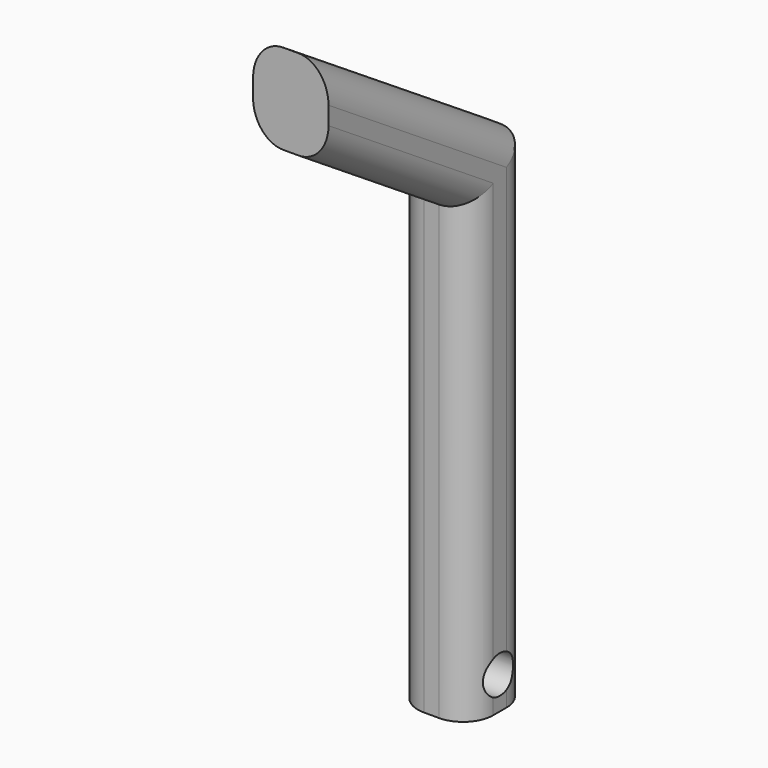
from build123d import *

# Parameters (mm, degrees)
F0_R         = 3.175
F1_DEPTH     = 12.7
F3_DEPTH     = 12.701
F4_T1_DEPTH  = 108.2499657273
F4_T3_DEPTH  = 76.2
F4_T8_DEPTH  = 101.5317029417
F4_T13_DEPTH = 101.5317029417
F4_T18_DEPTH = 60.7438000865
F4_T23_DEPTH = 60.7438000865
F4_T29_DEPTH = 101.5317029417
F4_T33_DEPTH = 60.7438000865
F4_T40_DEPTH = 101.5317029417
F4_T44_DEPTH = 60.7438000865


# Not quite as in the source:
# - a fillet or chamfer that OpenCascade refuses, or shapes differently, is made with other operations: its cross-section is extruded or revolved along the edge and cut away or added


with BuildPart() as f1:
    # F0 (on Right) → F1 (new body)
    with BuildSketch(Plane.YZ):
        Polygon((-12.9443686455, 18.7500342727), (0, 18.7500342727), (0, 101.6), (-42.5443466617, 129.3600174195), (-49.4843510166, 118.7239307541), (-12.9443686455, 94.8817372144), align=None)
        with Locations((-6.4721843228, 24.2384169251)):
            Circle(F0_R, mode=Mode.SUBTRACT)
    extrude(amount=F1_DEPTH)

    # F2 (on face) → F3 (cut, through all)
    with BuildSketch(Plane(origin=(0, 0, 0), x_dir=(0, -1, 0), z_dir=(-1, 0, 0))):
        Polygon((49.4843510166, 118.7239307541), (42.5443466617, 129.3600174195), (42.5443466617, 114.1956054441), align=None)
    extrude(amount=-F3_DEPTH, mode=Mode.SUBTRACT)

    # F4: fillet of radius 5.08 on 8 edges, made by hand

    # F4_s2 → F4_t1 (cut)
    with BuildSketch(Plane.XY.offset(6.0500342727)):
        with BuildLine():
            ThreePointArc((0, -5.08), (1.4878975516, -1.4878975516), (5.08, 0))
            Line((5.08, 0), (0, 0))
            Line((0, 0), (0, -5.08))
        make_face()
        with BuildLine():
            ThreePointArc((12.7, -5.08), (11.2121024484, -1.4878975516), (7.62, 0))
            Line((7.62, 0), (12.7, 0))
            Line((12.7, 0), (12.7, -5.08))
        make_face()
    extrude(amount=F4_T1_DEPTH, mode=Mode.SUBTRACT)

    # F4_s4 → F4_t3 (cut)
    with BuildSketch(Plane(origin=(0, -35.8612284696, 23.3993093117), x_dir=(1, 0, 0), z_dir=(0, -0.837487139, 0.5464570358))):
        with BuildLine():
            ThreePointArc((12.7, 80.0086933233), (11.2121024484, 83.6007957718), (7.62, 85.0886933233))
            Line((7.62, 85.0886933233), (12.7, 85.0886933233))
            Line((12.7, 85.0886933233), (12.7, 80.0086933233))
        make_face()
        with BuildLine():
            ThreePointArc((0, 80.0086933233), (1.4878975516, 83.6007957718), (5.08, 85.0886933233))
            Line((5.08, 85.0886933233), (0, 85.0886933233))
            Line((0, 85.0886933233), (0, 80.0086933233))
        make_face()
    extrude(amount=F4_T3_DEPTH, mode=Mode.SUBTRACT)


with BuildPart() as f4_tool6:
    # F4_s7 → F4_t8 (new body)
    with BuildSketch(Plane.XY.offset(107.5817372144)):
        with BuildLine():
            ThreePointArc((5.08, -12.9443686455), (1.4878975516, -11.456471094), (0, -7.8643686455))
            Line((0, -7.8643686455), (0, -12.9443686455))
            Line((0, -12.9443686455), (5.08, -12.9443686455))
        make_face()
    extrude(amount=-F4_T8_DEPTH)

    split(bisect_by=Plane(origin=(0, 39.5573107801, 60.624599668), x_dir=(1, 0, 0), z_dir=(0, -0.5464570358, -0.837487139)), keep=Keep.TOP)


with BuildPart() as f1_1:
    add(f1.part)

    # F4_t5: cut F4_tool6
    add(f4_tool6.part, mode=Mode.SUBTRACT)


with BuildPart() as f4_tool11:
    # F4_s12 → F4_t13 (new body)
    with BuildSketch(Plane.XY.offset(107.5817372144)):
        with BuildLine():
            ThreePointArc((7.62, -12.9443686455), (11.2121024484, -11.456471094), (12.7, -7.8643686455))
            Line((12.7, -7.8643686455), (12.7, -12.9443686455))
            Line((12.7, -12.9443686455), (7.62, -12.9443686455))
        make_face()
    extrude(amount=-F4_T13_DEPTH)

    split(bisect_by=Plane(origin=(0, 39.5573107801, 60.624599668), x_dir=(1, 0, 0), z_dir=(0, -0.5464570358, -0.837487139)), keep=Keep.TOP)


with BuildPart() as f1_2:
    add(f1_1.part)

    # F4_t10: cut F4_tool11
    add(f4_tool11.part, mode=Mode.SUBTRACT)


with BuildPart() as f4_tool16:
    # F4_s17 → F4_t18 (new body)
    with BuildSketch(Plane(origin=(0, -92.7377441072, 60.511010131), x_dir=(1, 0, 0), z_dir=(0, 0.837487139, -0.5464570358))):
        with BuildLine():
            ThreePointArc((7.62, -72.3886933233), (11.2121024484, -73.8765908749), (12.7, -77.4686933233))
            Line((12.7, -77.4686933233), (12.7, -72.3886933233))
            Line((12.7, -72.3886933233), (7.62, -72.3886933233))
        make_face()
    extrude(amount=F4_T18_DEPTH)

    split(bisect_by=Plane.XZ.offset(12.9443686455), keep=Keep.TOP)


with BuildPart() as f1_3:
    add(f1_2.part)

    # F4_t15: cut F4_tool16
    add(f4_tool16.part, mode=Mode.SUBTRACT)


with BuildPart() as f4_tool21:
    # F4_s22 → F4_t23 (new body)
    with BuildSketch(Plane(origin=(0, -92.7377441072, 60.511010131), x_dir=(1, 0, 0), z_dir=(0, 0.837487139, -0.5464570358))):
        with BuildLine():
            ThreePointArc((5.08, -72.3886933233), (1.4878975516, -73.8765908749), (0, -77.4686933233))
            Line((0, -77.4686933233), (0, -72.3886933233))
            Line((0, -72.3886933233), (5.08, -72.3886933233))
        make_face()
    extrude(amount=F4_T23_DEPTH)

    split(bisect_by=Plane.XZ.offset(12.9443686455), keep=Keep.TOP)


with BuildPart() as f1_4:
    add(f1_3.part)

    # F4_t20: cut F4_tool21
    add(f4_tool21.part, mode=Mode.SUBTRACT)


with BuildPart() as f4_tool27:
    # F4_s28 → F4_t29 (new body)
    with BuildSketch(Plane.XY.offset(107.5817372144)):
        with BuildLine():
            ThreePointArc((5.08, -12.9443686455), (1.4878975516, -11.456471094), (0, -7.8643686455))
            Line((0, -7.8643686455), (0, -12.9443686455))
            Line((0, -12.9443686455), (5.08, -12.9443686455))
        make_face()
    extrude(amount=-F4_T29_DEPTH)

    split(bisect_by=Plane(origin=(0, 39.5573107801, 60.624599668), x_dir=(1, 0, 0), z_dir=(0, 0.5464570358, 0.837487139)), keep=Keep.TOP)


with BuildPart() as f4_tool31:
    # F4_s32 → F4_t33 (new body)
    with BuildSketch(Plane(origin=(0, -92.7377441072, 60.511010131), x_dir=(1, 0, 0), z_dir=(0, 0.837487139, -0.5464570358))):
        with BuildLine():
            ThreePointArc((5.08, -72.3886933233), (1.4878975516, -73.8765908749), (0, -77.4686933233))
            Line((0, -77.4686933233), (0, -72.3886933233))
            Line((0, -72.3886933233), (5.08, -72.3886933233))
        make_face()
    extrude(amount=F4_T33_DEPTH)

    split(bisect_by=Plane.XZ.offset(12.9443686455), keep=Keep.BOTTOM)


with BuildPart() as f4_tool27_1:
    add(f4_tool27.part)

    # F4_t35: intersect F4_tool31
    add(f4_tool31.part, mode=Mode.INTERSECT)


with BuildPart() as f1_5:
    add(f1_4.part)

    # F4_t25: cut F4_tool27
    add(f4_tool27_1.part, mode=Mode.SUBTRACT)


with BuildPart() as f4_tool38:
    # F4_s39 → F4_t40 (new body)
    with BuildSketch(Plane.XY.offset(107.5817372144)):
        with BuildLine():
            ThreePointArc((7.62, -12.9443686455), (11.2121024484, -11.456471094), (12.7, -7.8643686455))
            Line((12.7, -7.8643686455), (12.7, -12.9443686455))
            Line((12.7, -12.9443686455), (7.62, -12.9443686455))
        make_face()
    extrude(amount=-F4_T40_DEPTH)

    split(bisect_by=Plane(origin=(0, 39.5573107801, 60.624599668), x_dir=(1, 0, 0), z_dir=(0, 0.5464570358, 0.837487139)), keep=Keep.TOP)


with BuildPart() as f4_tool42:
    # F4_s43 → F4_t44 (new body)
    with BuildSketch(Plane(origin=(0, -92.7377441072, 60.511010131), x_dir=(1, 0, 0), z_dir=(0, 0.837487139, -0.5464570358))):
        with BuildLine():
            ThreePointArc((7.62, -72.3886933233), (11.2121024484, -73.8765908749), (12.7, -77.4686933233))
            Line((12.7, -77.4686933233), (12.7, -72.3886933233))
            Line((12.7, -72.3886933233), (7.62, -72.3886933233))
        make_face()
    extrude(amount=F4_T44_DEPTH)

    split(bisect_by=Plane.XZ.offset(12.9443686455), keep=Keep.BOTTOM)


with BuildPart() as f4_tool38_1:
    add(f4_tool38.part)

    # F4_t46: intersect F4_tool42
    add(f4_tool42.part, mode=Mode.INTERSECT)


with BuildPart() as f1_6:
    add(f1_5.part)

    # F4_t36: cut F4_tool38
    add(f4_tool38_1.part, mode=Mode.SUBTRACT)


solid = f1_6.part
